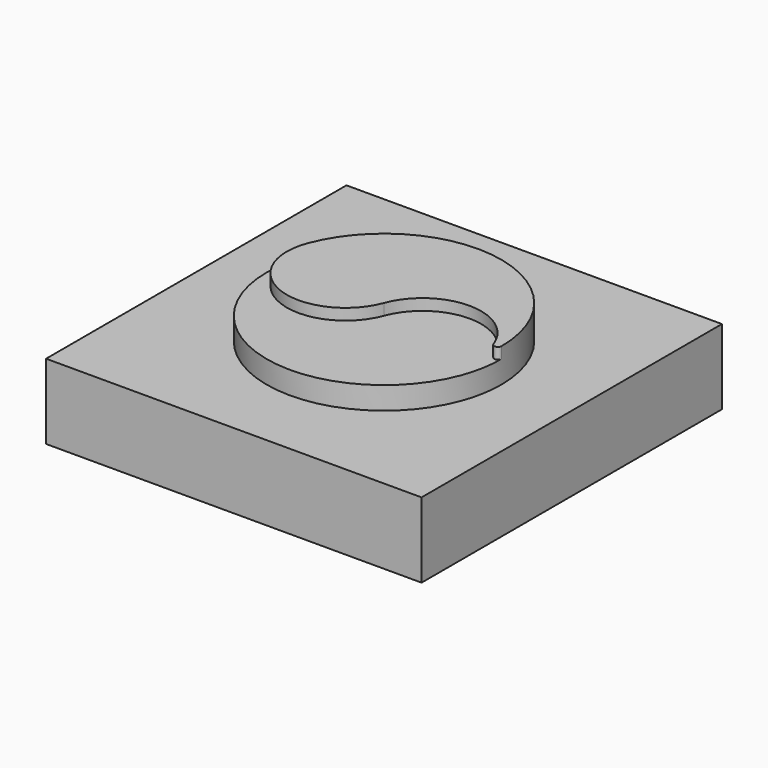
from build123d import *

# Parameters (mm, degrees)
F0_W        = 200
F0_H        = 200
F1_DEPTH    = 40
F3_DEPTH    = 12
F4_DEPTH    = 18
F5_T1_DEPTH = 62.2240943671


# Not quite as in the source:
# - a fillet or chamfer that OpenCascade refuses, or shapes differently, is made with other operations: its cross-section is extruded or revolved along the edge and cut away or added


with BuildPart() as f1:
    # F0 (on Top) → F1 (new body)
    with BuildSketch(Plane.XY):
        with Locations((-2.2933091968, 13.0733736824)):
            Rectangle(F0_W, F0_H)
    extrude(amount=F1_DEPTH)

    # F2 (on face) → F3 (join)
    with BuildSketch(Plane.XY.offset(40)):
        with BuildLine():
            Line((56.2270847505, 13.0733736824), (60.1964650758, 13.0733736824))
            ThreePointArc((60.1964650758, 13.0733736824), (8.8432450397, 74.5627959303), (-60.8137031442, 34.9899286326))
            ThreePointArc((-60.8137031442, 34.9899286326), (-62.7983933068, 24.0316511575), (-60.8137031442, 13.0733736824))
            Line((-60.8137031442, 13.0733736824), (-2.2933091968, 13.0733736824))
            ThreePointArc((-2.2933091968, 13.0733736824), (26.9668877768, 33.3599833436), (56.2270847505, 13.0733736824))
        make_face()
        with BuildLine():
            Line((-2.2933091968, 13.0733736824), (-60.8137031442, 13.0733736824))
            ThreePointArc((-60.8137031442, 13.0733736824), (-31.5535061705, -7.2132359788), (-2.2933091968, 13.0733736824))
        make_face()
        with BuildLine():
            ThreePointArc((-64.7830834694, 13.0733736824), (-13.4298634334, -48.4160485655), (56.2270847505, -8.8431812678))
            ThreePointArc((56.2270847505, -8.8431812678), (58.2117749131, 2.1150962073), (56.2270847505, 13.0733736824))
            Line((56.2270847505, 13.0733736824), (-2.2933091968, 13.0733736824))
            ThreePointArc((-2.2933091968, 13.0733736824), (-31.5535061705, -7.2132359788), (-60.8137031442, 13.0733736824))
            Line((-60.8137031442, 13.0733736824), (-64.7830834694, 13.0733736824))
        make_face()
        with BuildLine():
            ThreePointArc((-60.8137031442, 13.0733736824), (-62.7983933068, 24.0316511575), (-60.8137031442, 34.9899286326))
            ThreePointArc((-60.8137031442, 34.9899286326), (-63.7827314447, 24.2099279189), (-64.7830834694, 13.0733736824))
            Line((-64.7830834694, 13.0733736824), (-60.8137031442, 13.0733736824))
        make_face()
        with BuildLine():
            Line((-2.2933091968, 13.0733736824), (56.2270847505, 13.0733736824))
            ThreePointArc((56.2270847505, 13.0733736824), (26.9668877768, 33.3599833436), (-2.2933091968, 13.0733736824))
        make_face()
        with BuildLine():
            ThreePointArc((56.2270847505, -8.8431812678), (59.196113051, 1.9368194459), (60.1964650758, 13.0733736824))
            Line((60.1964650758, 13.0733736824), (56.2270847505, 13.0733736824))
            ThreePointArc((56.2270847505, 13.0733736824), (58.2117749131, 2.1150962073), (56.2270847505, -8.8431812678))
        make_face()
    extrude(amount=F3_DEPTH)

    # F2 (on face) → F4 (join)
    with BuildSketch(Plane.XY.offset(40)):
        with BuildLine():
            Line((56.2270847505, 13.0733736824), (60.1964650758, 13.0733736824))
            ThreePointArc((60.1964650758, 13.0733736824), (8.8432450397, 74.5627959303), (-60.8137031442, 34.9899286326))
            ThreePointArc((-60.8137031442, 34.9899286326), (-62.7983933068, 24.0316511575), (-60.8137031442, 13.0733736824))
            Line((-60.8137031442, 13.0733736824), (-2.2933091968, 13.0733736824))
            ThreePointArc((-2.2933091968, 13.0733736824), (26.9668877768, 33.3599833436), (56.2270847505, 13.0733736824))
        make_face()
        with BuildLine():
            Line((-2.2933091968, 13.0733736824), (-60.8137031442, 13.0733736824))
            ThreePointArc((-60.8137031442, 13.0733736824), (-31.5535061705, -7.2132359788), (-2.2933091968, 13.0733736824))
        make_face()
        with BuildLine():
            ThreePointArc((56.2270847505, -8.8431812678), (59.196113051, 1.9368194459), (60.1964650758, 13.0733736824))
            Line((60.1964650758, 13.0733736824), (56.2270847505, 13.0733736824))
            ThreePointArc((56.2270847505, 13.0733736824), (58.2117749131, 2.1150962073), (56.2270847505, -8.8431812678))
        make_face()
    extrude(amount=F4_DEPTH)

    # F5: fillet of radius 1.96 on 2 edges, made by hand

    # F5_s2 → F5_t1 (cut)
    with BuildSketch(Plane.XY.offset(52)):
        with BuildLine():
            ThreePointArc((60.196077506, 13.2934603584), (58.5741142709, 11.3559254547), (56.3903482373, 12.627134387))
            ThreePointArc((56.3903482373, 12.627134387), (58.2108716144, 1.8775122879), (56.2270847505, -8.8431812678))
            ThreePointArc((56.2270847505, -8.8431812678), (59.2156290063, 2.0451186179), (60.196077506, 13.2934603584))
        make_face()
    extrude(amount=F5_T1_DEPTH, mode=Mode.SUBTRACT)


solid = f1.part
